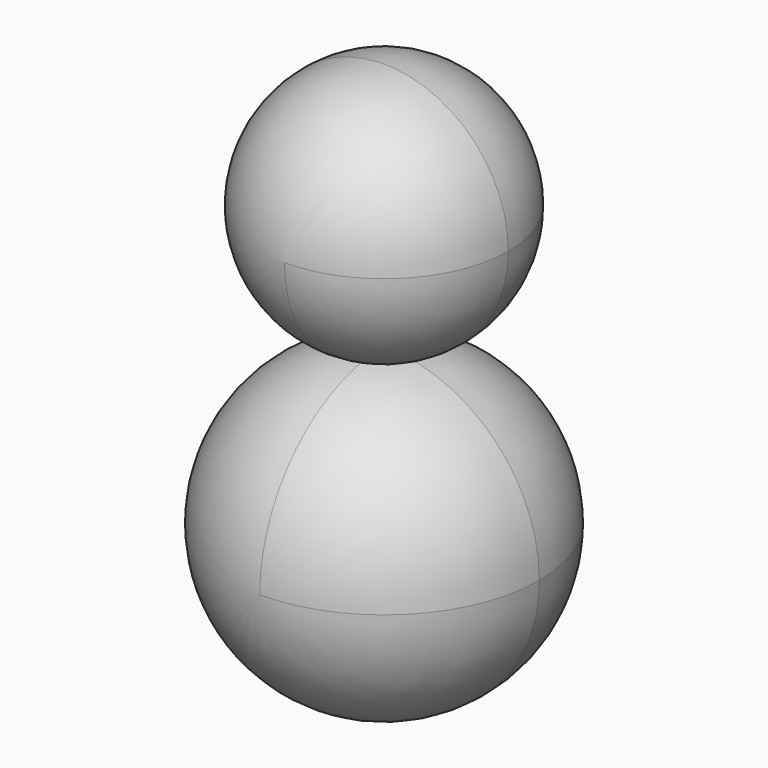
from build123d import *

# Parameters (mm, degrees)
F1_DEPTH      = 5
F1_DEPTH_BACK = 5
F2_R          = 4.99999
F3_DEPTH      = 4
F3_DEPTH_BACK = 4
F4_R          = 3.99999


# Not quite as in the source:
# - a fillet or chamfer is up to 0.001 mm smaller than in the source, because OpenCascade refuses the exact size


with BuildPart() as f1:
    # F0 (on Front) → F1 (new body, two sides)
    with BuildSketch(Plane.XZ) as f1_sk:
        with BuildLine():
            ThreePointArc((2.8e-09, 5), (-3.5355339069, -3.5355339049), (5, 0))
            ThreePointArc((5, 0), (3.5355339069, 3.5355339049), (2.8e-09, 5))
        make_face()
    extrude(amount=F1_DEPTH)
    extrude(f1_sk.sketch, amount=-F1_DEPTH_BACK)

    # F2 (radius 5 in the source; OpenCascade refuses exactly that, so slightly less here)
    f2_edges = [f1.edges().sort_by_distance(p)[0] for p in [
        (-5, -5, 0),
        (-5, 5, 0),
    ]]
    fillet(f2_edges, radius=F2_R)


with BuildPart() as f3:
    # F0 (on Front) → F3 (new body, two sides)
    with BuildSketch(Plane.XZ) as f3_sk:
        with BuildLine():
            ThreePointArc((4, 9), (-2.8284271257, 11.8284271237), (2.8e-09, 5))
            ThreePointArc((2.8e-09, 5), (2.8284271257, 6.1715728763), (4, 9))
        make_face()
    extrude(amount=F3_DEPTH)
    extrude(f3_sk.sketch, amount=-F3_DEPTH_BACK)

    # F4 (radius 4 in the source; OpenCascade refuses exactly that, so slightly less here)
    f4_edges = [f3.edges().sort_by_distance(p)[0] for p in [
        (0, 4, 13),
        (0, -4, 13),
    ]]
    fillet(f4_edges, radius=F4_R)


solid = Compound([f1.part, f3.part])
